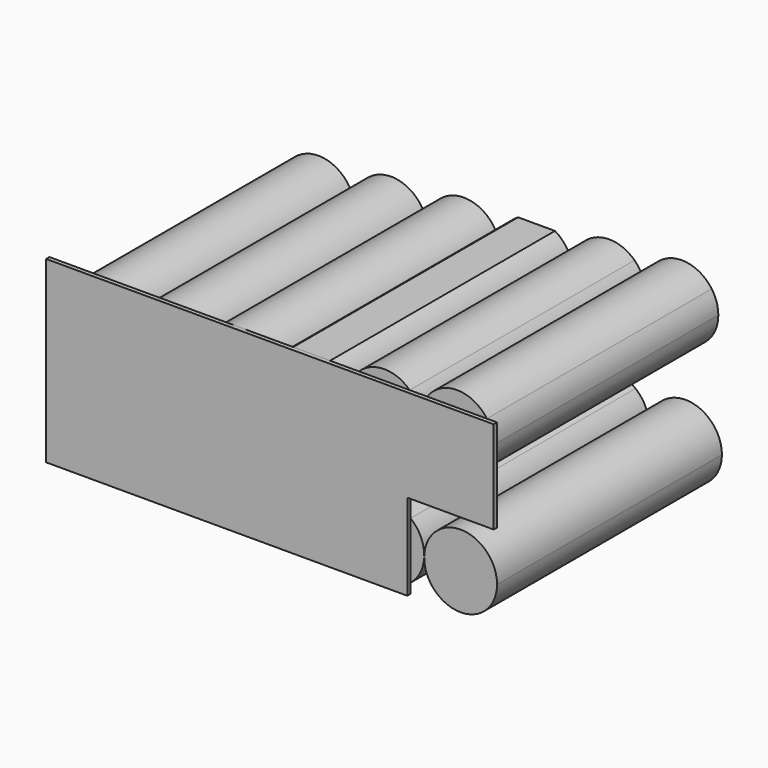
from build123d import *

# Parameters (mm, degrees)
F1_DEPTH = 4
F2_DEPTH = 270


with BuildPart() as f1:
    # F0 (on Front) → F1 (new body)
    with BuildSketch(Plane.XZ):
        with BuildLine():
            Line((-195.7849764046, 172), (-430, 172))
            Line((-430, 172), (-430, 25))
            Line((-430, 25), (-386.7711960698, 21.8855328581))
            ThreePointArc((-386.7711960698, 21.8855328581), (-419.2533574917, 57.2332605199), (-385.8963182023, 91.7565945325))
            ThreePointArc((-385.8963182023, 91.7565945325), (-413.7108642591, 149.9539874789), (-352.6270210914, 129.2332340666))
            ThreePointArc((-352.6270210914, 129.2332340666), (-320.2326008573, 166.6578457159), (-282.8079894646, 134.2634251853))
            ThreePointArc((-282.8079894646, 134.2634251853), (-250.4135683653, 171.6880353767), (-212.9889577288, 139.2936147916))
            ThreePointArc((-212.9889577288, 139.2936147916), (-209.055445323, 158.102487295), (-195.7849764046, 172))
        make_face()
        with BuildLine():
            Line((-160.373907248, 172), (-195.7849764046, 172))
            ThreePointArc((-195.7849764046, 172), (-209.055445323, 158.102487295), (-212.9889577288, 139.2936147916))
            ThreePointArc((-212.9889577288, 139.2936147916), (-200.9857572933, 115.3455136972), (-175.5643482834, 106.8991931564))
            ThreePointArc((-175.5643482834, 106.8991931564), (-152.4569100037, 117.9657675391), (-143.0794418263, 141.8087091151))
            ThreePointArc((-143.0794418263, 141.8087091151), (-143.1020701829, 143.0670703178), (-143.169925993, 144.3238043979))
            ThreePointArc((-143.169925993, 144.3238043979), (-148.3543878616, 160.286294639), (-160.373907248, 172))
        make_face()
        Polygon((-386.7711960698, 21.8855328581), (-430, 25), (-430, 0), (-83, 0), (-107.4950686991, 1.764774402), (-177.3141012878, 6.7949640697), (-247.1331326016, 11.8251536457), (-316.9521645982, 16.8553432708), align=None)
        with BuildLine():
            Line((-132.5897952544, 172), (-160.373907248, 172))
            ThreePointArc((-160.373907248, 172), (-148.3543878616, 160.286294639), (-143.169925993, 144.3238043979))
            ThreePointArc((-143.169925993, 144.3238043979), (-140.9529902982, 159.3367065037), (-132.5897952544, 172))
        make_face()
        with BuildLine():
            ThreePointArc((-175.5643482834, 106.8991931564), (-200.9857572933, 115.3455136972), (-212.9889577288, 139.2936147916))
            ThreePointArc((-212.9889577288, 139.2936147916), (-212.9211019187, 138.0368807115), (-212.8984735621, 136.7785195088))
            ThreePointArc((-212.8984735621, 136.7785195088), (-222.2759410866, 112.9355786344), (-245.3833781073, 101.8690036878))
            Line((-245.3833781073, 101.8690036878), (-175.5643482834, 106.8991931564))
        make_face()
        with BuildLine():
            ThreePointArc((-212.8984735621, 136.7785195088), (-212.9211019187, 138.0368807115), (-212.9889577288, 139.2936147916))
            ThreePointArc((-212.9889577288, 139.2936147916), (-250.4135683653, 171.6880353767), (-282.8079894646, 134.2634251853))
            ThreePointArc((-282.8079894646, 134.2634251853), (-270.8047883044, 110.3153234636), (-245.3833781073, 101.8690036878))
            ThreePointArc((-245.3833781073, 101.8690036878), (-222.2759410866, 112.9355786344), (-212.8984735621, 136.7785195088))
        make_face()
        with BuildLine():
            ThreePointArc((-349.3465849767, 54.2799543745), (-361.3497860368, 30.3318527395), (-386.7711960698, 21.8855328581))
            Line((-386.7711960698, 21.8855328581), (-316.9521645982, 16.8553432708))
            ThreePointArc((-316.9521645982, 16.8553432708), (-340.9002655033, 28.858544713), (-349.3465849767, 54.2799543745))
        make_face()
        with BuildLine():
            ThreePointArc((-385.8963182023, 91.7565945325), (-419.2533574917, 57.2332605199), (-386.7711960698, 21.8855328581))
            ThreePointArc((-386.7711960698, 21.8855328581), (-361.3497860368, 30.3318527395), (-349.3465849767, 54.2799543745))
            ThreePointArc((-349.3465849767, 54.2799543745), (-349.2787292185, 55.5366879759), (-349.2561008792, 56.795048698))
            ThreePointArc((-349.2561008792, 56.795048698), (-360.0942260172, 82.1170510508), (-385.8963182023, 91.7565945325))
        make_face()
        with BuildLine():
            Line((-83.9310249267, 172), (-132.5897952544, 172))
            ThreePointArc((-132.5897952544, 172), (-140.9529902982, 159.3367065037), (-143.169925993, 144.3238043979))
            ThreePointArc((-143.169925993, 144.3238043979), (-131.166725929, 120.3757036251), (-105.7453175279, 111.9293826921))
            ThreePointArc((-105.7453175279, 111.9293826921), (-82.6378786027, 122.9959567856), (-73.2604100905, 146.8388987214))
            ThreePointArc((-73.2604100905, 146.8388987214), (-73.2830384471, 148.0972599242), (-73.3508942572, 149.3539940042))
            ThreePointArc((-73.3508942572, 149.3539940042), (-76.5504393443, 161.6536803692), (-83.9310249267, 172))
        make_face()
        with BuildLine():
            ThreePointArc((-105.7453175279, 111.9293826921), (-131.166725929, 120.3757036251), (-143.169925993, 144.3238043979))
            ThreePointArc((-143.169925993, 144.3238043979), (-143.1020701829, 143.0670703178), (-143.0794418263, 141.8087091151))
            ThreePointArc((-143.0794418263, 141.8087091151), (-152.4569100037, 117.9657675391), (-175.5643482834, 106.8991931564))
            Line((-175.5643482834, 106.8991931564), (-105.7453175279, 111.9293826921))
        make_face()
        with BuildLine():
            ThreePointArc((-245.3833781073, 101.8690036878), (-270.8047883044, 110.3153234636), (-282.8079894646, 134.2634251853))
            ThreePointArc((-282.8079894646, 134.2634251853), (-282.7401336545, 133.0066911052), (-282.7175052979, 131.7483299025))
            ThreePointArc((-282.7175052979, 131.7483299025), (-292.0949733471, 107.9053884642), (-315.2024113796, 96.8388139708))
            Line((-315.2024113796, 96.8388139708), (-245.3833781073, 101.8690036878))
        make_face()
        with BuildLine():
            ThreePointArc((-282.7175052979, 131.7483299025), (-282.7401336545, 133.0066911052), (-282.8079894646, 134.2634251853))
            ThreePointArc((-282.8079894646, 134.2634251853), (-320.2326008573, 166.6578457159), (-352.6270210914, 129.2332340666))
            ThreePointArc((-352.6270210914, 129.2332340666), (-340.6238200494, 105.2851338652), (-315.2024113796, 96.8388139708))
            ThreePointArc((-315.2024113796, 96.8388139708), (-292.0949733471, 107.9053884642), (-282.7175052979, 131.7483299025))
        make_face()
        with BuildLine():
            Line((-105.7453175279, 111.9293826921), (-175.5643482834, 106.8991931564))
            Line((-175.5643482834, 106.8991931564), (-245.3833781073, 101.8690036878))
            Line((-245.3833781073, 101.8690036878), (-315.2024113796, 96.8388139708))
            ThreePointArc((-315.2024113796, 96.8388139708), (-340.6238200494, 105.2851338652), (-352.6270210914, 129.2332340666))
            ThreePointArc((-352.6270210914, 129.2332340666), (-352.559165363, 127.9765007412), (-352.5365370337, 126.7181402961))
            ThreePointArc((-352.5365370337, 126.7181402961), (-362.2145341598, 102.5562659804), (-385.8963182023, 91.7565945325))
            ThreePointArc((-385.8963182023, 91.7565945325), (-360.0942260172, 82.1170510508), (-349.2561008792, 56.795048698))
            ThreePointArc((-349.2561008792, 56.795048698), (-349.2787292185, 55.5366879759), (-349.3465849767, 54.2799543745))
            ThreePointArc((-349.3465849767, 54.2799543745), (-313.1787079407, 86.7422307352), (-279.4370691434, 51.7648590917))
            ThreePointArc((-279.4370691434, 51.7648590917), (-279.4596974729, 50.5064986405), (-279.527553202, 49.249765309))
            ThreePointArc((-279.527553202, 49.249765309), (-243.359675934, 81.7120411191), (-209.6180374076, 46.7346694854))
            ThreePointArc((-209.6180374076, 46.7346694854), (-209.6406657369, 45.4763090403), (-209.7085214653, 44.2195757149))
            ThreePointArc((-209.7085214653, 44.2195757149), (-173.540644192, 76.6818515125), (-139.7990056718, 41.7044798791))
            ThreePointArc((-139.7990056718, 41.7044798791), (-139.8216340111, 40.4461191571), (-139.8894897693, 39.189385556))
            ThreePointArc((-139.8894897693, 39.189385556), (-118.9296132608, 68.7742523087), (-83, 63.9117781483))
            Line((-83, 63.9117781483), (-83, 83))
            Line((-83, 83), (0, 83))
            Line((0, 83), (0, 119.5479214189))
            Line((0, 119.5479214189), (-35.9262829, 116.9595725068))
            Line((-35.9262829, 116.9595725068), (-105.7453175279, 111.9293826921))
        make_face()
        with BuildLine():
            Line((-107.4950686991, 1.764774402), (-83, 0))
            Line((-83, 0), (-83, 9.4368023971))
            ThreePointArc((-83, 9.4368023971), (-94.5188371099, 3.2742211664), (-107.4950686991, 1.764774402))
        make_face()
        with BuildLine():
            ThreePointArc((-279.527553202, 49.249765309), (-291.5307541961, 25.3016632239), (-316.9521645982, 16.8553432708))
            Line((-316.9521645982, 16.8553432708), (-247.1331326016, 11.8251536457))
            ThreePointArc((-247.1331326016, 11.8251536457), (-271.0812338594, 23.8283552128), (-279.527553202, 49.249765309))
        make_face()
        with BuildLine():
            ThreePointArc((-349.3465849767, 54.2799543745), (-340.9002655033, 28.858544713), (-316.9521645982, 16.8553432708))
            ThreePointArc((-316.9521645982, 16.8553432708), (-291.5307541961, 25.3016632239), (-279.527553202, 49.249765309))
            ThreePointArc((-279.527553202, 49.249765309), (-279.4596974729, 50.5064986405), (-279.4370691434, 51.7648590917))
            ThreePointArc((-279.4370691434, 51.7648590917), (-313.1787079407, 86.7422307352), (-349.3465849767, 54.2799543745))
        make_face()
        with BuildLine():
            ThreePointArc((-352.6270210914, 129.2332340666), (-413.7108642591, 149.9539874789), (-385.8963182023, 91.7565945325))
            ThreePointArc((-385.8963182023, 91.7565945325), (-362.2145341598, 102.5562659804), (-352.5365370337, 126.7181402961))
            ThreePointArc((-352.5365370337, 126.7181402961), (-352.559165363, 127.9765007412), (-352.6270210914, 129.2332340666))
        make_face()
        with BuildLine():
            Line((-67.0725920077, 172), (-83.9310249267, 172))
            ThreePointArc((-83.9310249267, 172), (-76.5504393443, 161.6536803692), (-73.3508942572, 149.3539940042))
            ThreePointArc((-73.3508942572, 149.3539940042), (-72.1692077394, 161.2196778814), (-67.0725920077, 172))
        make_face()
        with BuildLine():
            ThreePointArc((-73.2604100905, 146.8388987214), (-82.6378786027, 122.9959567856), (-105.7453175279, 111.9293826921))
            Line((-105.7453175279, 111.9293826921), (-35.9262829, 116.9595725068))
            ThreePointArc((-35.9262829, 116.9595725068), (-61.347693097, 125.4058922826), (-73.3508942572, 149.3539940042))
            ThreePointArc((-73.3508942572, 149.3539940042), (-73.2830384471, 148.0972599242), (-73.2604100905, 146.8388987214))
        make_face()
        with BuildLine():
            Line((-177.3141012878, 6.7949640697), (-107.4950686991, 1.764774402))
            ThreePointArc((-107.4950686991, 1.764774402), (-131.4431700691, 13.767975632), (-139.8894897693, 39.189385556))
            ThreePointArc((-139.8894897693, 39.189385556), (-151.8926909904, 15.2412837811), (-177.3141012878, 6.7949640697))
        make_face()
        with BuildLine():
            ThreePointArc((-139.8894897693, 39.189385556), (-131.4431700691, 13.767975632), (-107.4950686991, 1.764774402))
            ThreePointArc((-107.4950686991, 1.764774402), (-94.5188371099, 3.2742211664), (-83, 9.4368023971))
            Line((-83, 9.4368023971), (-83, 63.9117781483))
            ThreePointArc((-83, 63.9117781483), (-118.9296132608, 68.7742523087), (-139.8894897693, 39.189385556))
        make_face()
        with BuildLine():
            ThreePointArc((-279.527553202, 49.249765309), (-271.0812338594, 23.8283552128), (-247.1331326016, 11.8251536457))
            ThreePointArc((-247.1331326016, 11.8251536457), (-221.7117223568, 20.2714737072), (-209.7085214653, 44.2195757149))
            ThreePointArc((-209.7085214653, 44.2195757149), (-209.6406657369, 45.4763090403), (-209.6180374076, 46.7346694854))
            ThreePointArc((-209.6180374076, 46.7346694854), (-243.359675934, 81.7120411191), (-279.527553202, 49.249765309))
        make_face()
        with BuildLine():
            ThreePointArc((-209.7085214653, 44.2195757149), (-221.7117223568, 20.2714737072), (-247.1331326016, 11.8251536457))
            Line((-247.1331326016, 11.8251536457), (-177.3141012878, 6.7949640697))
            ThreePointArc((-177.3141012878, 6.7949640697), (-201.2622022661, 18.7981657711), (-209.7085214653, 44.2195757149))
        make_face()
        with BuildLine():
            Line((-9.8101647017, 172), (-67.0725920077, 172))
            ThreePointArc((-67.0725920077, 172), (-72.1692077394, 161.2196778814), (-73.3508942572, 149.3539940042))
            ThreePointArc((-73.3508942572, 149.3539940042), (-61.347693097, 125.4058922826), (-35.9262829, 116.9595725068))
            ThreePointArc((-35.9262829, 116.9595725068), (-12.8188458792, 128.0261474533), (-3.4413783547, 151.8690883278))
            ThreePointArc((-3.4413783547, 151.8690883278), (-5.0715380955, 162.426254665), (-9.8101647017, 172))
        make_face()
        with BuildLine():
            ThreePointArc((-3.4413783547, 151.8690883278), (-12.8188458792, 128.0261474533), (-35.9262829, 116.9595725068))
            Line((-35.9262829, 116.9595725068), (0, 119.5479214189))
            Line((0, 119.5479214189), (0, 172))
            Line((0, 172), (-9.8101647017, 172))
            ThreePointArc((-9.8101647017, 172), (-5.0715380955, 162.426254665), (-3.4413783547, 151.8690883278))
        make_face()
        with BuildLine():
            ThreePointArc((-177.3141012878, 6.7949640697), (-151.8926909904, 15.2412837811), (-139.8894897693, 39.189385556))
            ThreePointArc((-139.8894897693, 39.189385556), (-139.8216340111, 40.4461191571), (-139.7990056718, 41.7044798791))
            ThreePointArc((-139.7990056718, 41.7044798791), (-173.540644192, 76.6818515125), (-209.7085214653, 44.2195757149))
            ThreePointArc((-209.7085214653, 44.2195757149), (-201.2622022661, 18.7981657711), (-177.3141012878, 6.7949640697))
        make_face()
    extrude(amount=F1_DEPTH)


with BuildPart() as f2:
    # F0 (on Front) → F2 (new body)
    with BuildSketch(Plane.XZ):
        with BuildLine():
            ThreePointArc((-385.8963182023, 91.7565945325), (-419.2533574917, 57.2332605199), (-386.7711960698, 21.8855328581))
            ThreePointArc((-386.7711960698, 21.8855328581), (-361.3497860368, 30.3318527395), (-349.3465849767, 54.2799543745))
            ThreePointArc((-349.3465849767, 54.2799543745), (-349.2787292185, 55.5366879759), (-349.2561008792, 56.795048698))
            ThreePointArc((-349.2561008792, 56.795048698), (-360.0942260172, 82.1170510508), (-385.8963182023, 91.7565945325))
        make_face()
    extrude(amount=-F2_DEPTH)


with BuildPart() as f2b:
    # F0 (on Front) → F2, piece 2 (new body)
    with BuildSketch(Plane.XZ):
        with BuildLine():
            ThreePointArc((-349.3465849767, 54.2799543745), (-340.9002655033, 28.858544713), (-316.9521645982, 16.8553432708))
            ThreePointArc((-316.9521645982, 16.8553432708), (-291.5307541961, 25.3016632239), (-279.527553202, 49.249765309))
            ThreePointArc((-279.527553202, 49.249765309), (-279.4596974729, 50.5064986405), (-279.4370691434, 51.7648590917))
            ThreePointArc((-279.4370691434, 51.7648590917), (-313.1787079407, 86.7422307352), (-349.3465849767, 54.2799543745))
        make_face()
    extrude(amount=-F2_DEPTH)


with BuildPart() as f2c:
    # F0 (on Front) → F2, piece 3 (new body)
    with BuildSketch(Plane.XZ):
        with BuildLine():
            ThreePointArc((-279.527553202, 49.249765309), (-271.0812338594, 23.8283552128), (-247.1331326016, 11.8251536457))
            ThreePointArc((-247.1331326016, 11.8251536457), (-221.7117223568, 20.2714737072), (-209.7085214653, 44.2195757149))
            ThreePointArc((-209.7085214653, 44.2195757149), (-209.6406657369, 45.4763090403), (-209.6180374076, 46.7346694854))
            ThreePointArc((-209.6180374076, 46.7346694854), (-243.359675934, 81.7120411191), (-279.527553202, 49.249765309))
        make_face()
    extrude(amount=-F2_DEPTH)


with BuildPart() as f2d:
    # F0 (on Front) → F2, piece 4 (new body)
    with BuildSketch(Plane.XZ):
        with BuildLine():
            ThreePointArc((-177.3141012878, 6.7949640697), (-151.8926909904, 15.2412837811), (-139.8894897693, 39.189385556))
            ThreePointArc((-139.8894897693, 39.189385556), (-139.8216340111, 40.4461191571), (-139.7990056718, 41.7044798791))
            ThreePointArc((-139.7990056718, 41.7044798791), (-173.540644192, 76.6818515125), (-209.7085214653, 44.2195757149))
            ThreePointArc((-209.7085214653, 44.2195757149), (-201.2622022661, 18.7981657711), (-177.3141012878, 6.7949640697))
        make_face()
    extrude(amount=-F2_DEPTH)


with BuildPart() as f2e:
    # F0 (on Front) → F2, piece 5 (new body)
    with BuildSketch(Plane.XZ):
        with BuildLine():
            ThreePointArc((-139.8894897693, 39.189385556), (-131.4431700691, 13.767975632), (-107.4950686991, 1.764774402))
            ThreePointArc((-107.4950686991, 1.764774402), (-94.5188371099, 3.2742211664), (-83, 9.4368023971))
            Line((-83, 9.4368023971), (-83, 63.9117781483))
            ThreePointArc((-83, 63.9117781483), (-118.9296132608, 68.7742523087), (-139.8894897693, 39.189385556))
        make_face()
        with BuildLine():
            Line((-83, 63.9117781483), (-83, 9.4368023971))
            ThreePointArc((-83, 9.4368023971), (-73.5850916032, 21.2029825287), (-69.989986966, 35.8371452194))
            ThreePointArc((-69.989986966, 35.8371452194), (-69.982477283, 36.2556878059), (-69.979973936, 36.6742902727))
            ThreePointArc((-69.979973936, 36.6742902727), (-73.402299166, 51.7690064383), (-83, 63.9117781483))
        make_face()
    extrude(amount=-F2_DEPTH)


with BuildPart() as f2f:
    # F0 (on Front) → F2, piece 6 (new body)
    with BuildSketch(Plane.XZ):
        with BuildLine():
            ThreePointArc((-69.989986966, 35.8371452194), (-60.0429639642, 10.5490295512), (-35.0000001584, 0))
            ThreePointArc((-35.0000001584, 0), (-10.2512627145, 10.2512626025), (0, 35))
            ThreePointArc((0, 35), (-34.5813974501, 69.997496652), (-69.989986966, 35.8371452194))
        make_face()
    extrude(amount=-F2_DEPTH)


with BuildPart() as f2g:
    # F0 (on Front) → F2, piece 7 (new body)
    with BuildSketch(Plane.XZ):
        with BuildLine():
            Line((-9.8101647017, 172), (-67.0725920077, 172))
            ThreePointArc((-67.0725920077, 172), (-72.1692077394, 161.2196778814), (-73.3508942572, 149.3539940042))
            ThreePointArc((-73.3508942572, 149.3539940042), (-61.347693097, 125.4058922826), (-35.9262829, 116.9595725068))
            ThreePointArc((-35.9262829, 116.9595725068), (-12.8188458792, 128.0261474533), (-3.4413783547, 151.8690883278))
            ThreePointArc((-3.4413783547, 151.8690883278), (-5.0715380955, 162.426254665), (-9.8101647017, 172))
        make_face()
        with BuildLine():
            ThreePointArc((-9.8101647017, 172), (-38.4413783547, 186.8690883278), (-67.0725920077, 172))
            Line((-67.0725920077, 172), (-9.8101647017, 172))
        make_face()
    extrude(amount=-F2_DEPTH)


with BuildPart() as f2h:
    # F0 (on Front) → F2, piece 8 (new body)
    with BuildSketch(Plane.XZ):
        with BuildLine():
            Line((-160.373907248, 172), (-195.7849764046, 172))
            ThreePointArc((-195.7849764046, 172), (-209.055445323, 158.102487295), (-212.9889577288, 139.2936147916))
            ThreePointArc((-212.9889577288, 139.2936147916), (-200.9857572933, 115.3455136972), (-175.5643482834, 106.8991931564))
            ThreePointArc((-175.5643482834, 106.8991931564), (-152.4569100037, 117.9657675391), (-143.0794418263, 141.8087091151))
            ThreePointArc((-143.0794418263, 141.8087091151), (-143.1020701829, 143.0670703178), (-143.169925993, 144.3238043979))
            ThreePointArc((-143.169925993, 144.3238043979), (-148.3543878616, 160.286294639), (-160.373907248, 172))
        make_face()
    extrude(amount=-F2_DEPTH)


with BuildPart() as f2i:
    # F0 (on Front) → F2, piece 9 (new body)
    with BuildSketch(Plane.XZ):
        with BuildLine():
            ThreePointArc((-212.8984735621, 136.7785195088), (-212.9211019187, 138.0368807115), (-212.9889577288, 139.2936147916))
            ThreePointArc((-212.9889577288, 139.2936147916), (-250.4135683653, 171.6880353767), (-282.8079894646, 134.2634251853))
            ThreePointArc((-282.8079894646, 134.2634251853), (-270.8047883044, 110.3153234636), (-245.3833781073, 101.8690036878))
            ThreePointArc((-245.3833781073, 101.8690036878), (-222.2759410866, 112.9355786344), (-212.8984735621, 136.7785195088))
        make_face()
    extrude(amount=-F2_DEPTH)


with BuildPart() as f2j:
    # F0 (on Front) → F2, piece 10 (new body)
    with BuildSketch(Plane.XZ):
        with BuildLine():
            ThreePointArc((-282.7175052979, 131.7483299025), (-282.7401336545, 133.0066911052), (-282.8079894646, 134.2634251853))
            ThreePointArc((-282.8079894646, 134.2634251853), (-320.2326008573, 166.6578457159), (-352.6270210914, 129.2332340666))
            ThreePointArc((-352.6270210914, 129.2332340666), (-340.6238200494, 105.2851338652), (-315.2024113796, 96.8388139708))
            ThreePointArc((-315.2024113796, 96.8388139708), (-292.0949733471, 107.9053884642), (-282.7175052979, 131.7483299025))
        make_face()
    extrude(amount=-F2_DEPTH)


with BuildPart() as f2k:
    # F0 (on Front) → F2, piece 11 (new body)
    with BuildSketch(Plane.XZ):
        with BuildLine():
            ThreePointArc((-352.6270210914, 129.2332340666), (-413.7108642591, 149.9539874789), (-385.8963182023, 91.7565945325))
            ThreePointArc((-385.8963182023, 91.7565945325), (-362.2145341598, 102.5562659804), (-352.5365370337, 126.7181402961))
            ThreePointArc((-352.5365370337, 126.7181402961), (-352.559165363, 127.9765007412), (-352.6270210914, 129.2332340666))
        make_face()
    extrude(amount=-F2_DEPTH)


with BuildPart() as f2l:
    # F0 (on Front) → F2, piece 12 (new body)
    with BuildSketch(Plane.XZ):
        with BuildLine():
            Line((-83.9310249267, 172), (-132.5897952544, 172))
            ThreePointArc((-132.5897952544, 172), (-140.9529902982, 159.3367065037), (-143.169925993, 144.3238043979))
            ThreePointArc((-143.169925993, 144.3238043979), (-131.166725929, 120.3757036251), (-105.7453175279, 111.9293826921))
            ThreePointArc((-105.7453175279, 111.9293826921), (-82.6378786027, 122.9959567856), (-73.2604100905, 146.8388987214))
            ThreePointArc((-73.2604100905, 146.8388987214), (-73.2830384471, 148.0972599242), (-73.3508942572, 149.3539940042))
            ThreePointArc((-73.3508942572, 149.3539940042), (-76.5504393443, 161.6536803692), (-83.9310249267, 172))
        make_face()
        with BuildLine():
            ThreePointArc((-83.9310249267, 172), (-108.2604100905, 181.8388987214), (-132.5897952544, 172))
            Line((-132.5897952544, 172), (-83.9310249267, 172))
        make_face()
    extrude(amount=-F2_DEPTH)


solid = Compound([f1.part, f2.part, f2b.part, f2c.part, f2d.part, f2e.part, f2f.part, f2g.part, f2h.part, f2i.part, f2j.part, f2k.part, f2l.part])
